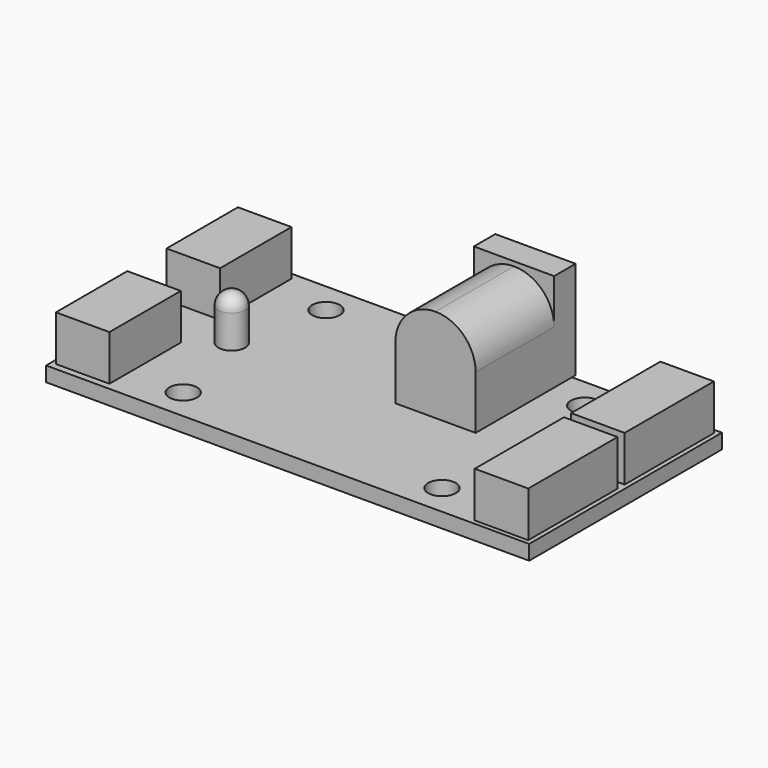
from build123d import *

# Parameters (mm, degrees)
F0_W      = 6
F0_H      = 10
F0_R      = 1.55
F0_R_2    = 1.5
F0_W_2    = 10
F0_H_2    = 22
F0_H_3    = 12.5
F0_W_3    = 9
F0_H_4    = 11
F0_H_5    = 2.5
F1_DEPTH  = 1.66
F0_H_6    = 0.5
F2_DEPTH  = 11
F3_DEPTH  = 10.5
F4_R      = 4.49999
F5_R      = 3.25
F6_DEPTH  = 10
F7_DEPTH  = 5.2
F8_R      = 1.5
F9_DEPTH  = 5.1
F10_W     = 1
F10_H     = 1
F11_DEPTH = 2.3


# Not quite as in the source:
# - a fillet or chamfer is up to 0.001 mm smaller than in the source, because OpenCascade refuses the exact size


with BuildPart() as f1:
    # F0 (on Top) → F1 (new body)
    with BuildSketch(Plane.XY):
        Polygon((-27.07, -13.5), (27.07, -13.5), (27.07, 13.5), (10.27, 13.5), (10.27, 11), (10.27, 0), (1.27, 0), (1.27, 11), (1.27, 13.5), (-27.07, 13.5), align=None)
        with Locations((-23.57, -7.75)):
            Rectangle(F0_W, F0_H, mode=Mode.SUBTRACT)
        with Locations((-14.5, -10)):
            Circle(F0_R, mode=Mode.SUBTRACT)
        with Locations((-17.07, 0)):
            Circle(F0_R_2, mode=Mode.SUBTRACT)
        with Locations((-6.07, 0)):
            Rectangle(F0_W_2, F0_H_2, mode=Mode.SUBTRACT)
        with Locations((14.5, -10)):
            Circle(F0_R, mode=Mode.SUBTRACT)
        with Locations((23.57, -6.75)):
            Rectangle(F0_W, F0_H_3, mode=Mode.SUBTRACT)
        with Locations((-23.57, 7.75)):
            Rectangle(F0_W, F0_H, mode=Mode.SUBTRACT)
        with Locations((-14.5, 10)):
            Circle(F0_R, mode=Mode.SUBTRACT)
        with Locations((23.57, 6.75)):
            Rectangle(F0_W, F0_H_3, mode=Mode.SUBTRACT)
        with Locations((14.5, 10)):
            Circle(F0_R, mode=Mode.SUBTRACT)
        with Locations((-6.07, 0)):
            Rectangle(F0_W_2, F0_H_2)
        with Locations((5.77, 5.5)):
            Rectangle(F0_W_3, F0_H_4)
        with Locations((23.57, 6.75)):
            Rectangle(F0_W, F0_H_3)
        with Locations((23.57, -6.75)):
            Rectangle(F0_W, F0_H_3)
        with Locations((-23.57, 7.75)):
            Rectangle(F0_W, F0_H)
        with Locations((-23.57, -7.75)):
            Rectangle(F0_W, F0_H)
        with Locations((5.77, 12.25)):
            Rectangle(F0_W_3, F0_H_5)
        with Locations((-17.07, 0)):
            Circle(F0_R_2)
    extrude(amount=-F1_DEPTH)

    # F0 (on Top) → F2 (join)
    with BuildSketch(Plane.XY):
        with Locations((5.77, 12.25)):
            Rectangle(F0_W_3, F0_H_5)
        with Locations((5.77, 13.75)):
            Rectangle(F0_W_3, F0_H_6)
    extrude(amount=F2_DEPTH)

    # F0 (on Top) → F3 (join)
    with BuildSketch(Plane.XY):
        with Locations((5.77, 5.5)):
            Rectangle(F0_W_3, F0_H_4)
    extrude(amount=F3_DEPTH)

    # F4 (radius 4.5 in the source; OpenCascade refuses exactly that, so slightly less here)
    f4_edges = [f1.edges().sort_by_distance(p)[0] for p in [
        (1.27, 5.5, 10.5),
        (10.27, 5.5, 10.5),
    ]]
    fillet(f4_edges, radius=F4_R)

    # F5 (on face) → F6 (cut)
    with BuildSketch(Plane(origin=(0, 14, 0), x_dir=(-1, 0, 0), z_dir=(0, 1, 0))):
        with Locations((-5.77, 6.3)):
            Circle(F5_R)
    extrude(amount=-F6_DEPTH, mode=Mode.SUBTRACT)

    # F0 (on Top) → F7 (join)
    with BuildSketch(Plane.XY):
        with Locations((-17.07, 0)):
            Circle(F0_R_2)
    extrude(amount=F7_DEPTH)

    # F8
    f8_edges = [f1.edges().sort_by_distance(p)[0] for p in [
        (-18.57, 0, 5.2),
    ]]
    fillet(f8_edges, radius=F8_R)

    # F0 (on Top) → F9 (join)
    with BuildSketch(Plane.XY):
        with Locations((23.57, 6.75)):
            Rectangle(F0_W, F0_H_3)
        with Locations((23.57, -6.75)):
            Rectangle(F0_W, F0_H_3)
        with Locations((-23.57, -7.75)):
            Rectangle(F0_W, F0_H)
        with Locations((-23.57, 7.75)):
            Rectangle(F0_W, F0_H)
    extrude(amount=F9_DEPTH)

    # F10 (on face) → F11 (join)
    with BuildSketch(Plane(origin=(0, 0, -1.66), x_dir=(1, 0, 0), z_dir=(0, 0, -1))):
        Rectangle(F10_W, F10_H)
        with Locations((0, 7)):
            Rectangle(F10_W, F10_H)
        with Locations((5.5, 7)):
            Rectangle(F10_W, F10_H)
        with Locations((11, 7)):
            Rectangle(F10_W, F10_H)
        with Locations((11, 0)):
            Rectangle(F10_W, F10_H)
        with Locations((5.5, 0)):
            Rectangle(F10_W, F10_H)
        with Locations((11, -7)):
            Rectangle(F10_W, F10_H)
        with Locations((5.5, -7)):
            Rectangle(F10_W, F10_H)
        with Locations((0, -7)):
            Rectangle(F10_W, F10_H)
        with Locations((-5.5, -7)):
            Rectangle(F10_W, F10_H)
        with Locations((-5.5, 0)):
            Rectangle(F10_W, F10_H)
        with Locations((-5.5, 7)):
            Rectangle(F10_W, F10_H)
        with Locations((-11, 7)):
            Rectangle(F10_W, F10_H)
        with Locations((-11, 0)):
            Rectangle(F10_W, F10_H)
        with Locations((-11, -7)):
            Rectangle(F10_W, F10_H)
    extrude(amount=F11_DEPTH)


solid = f1.part
